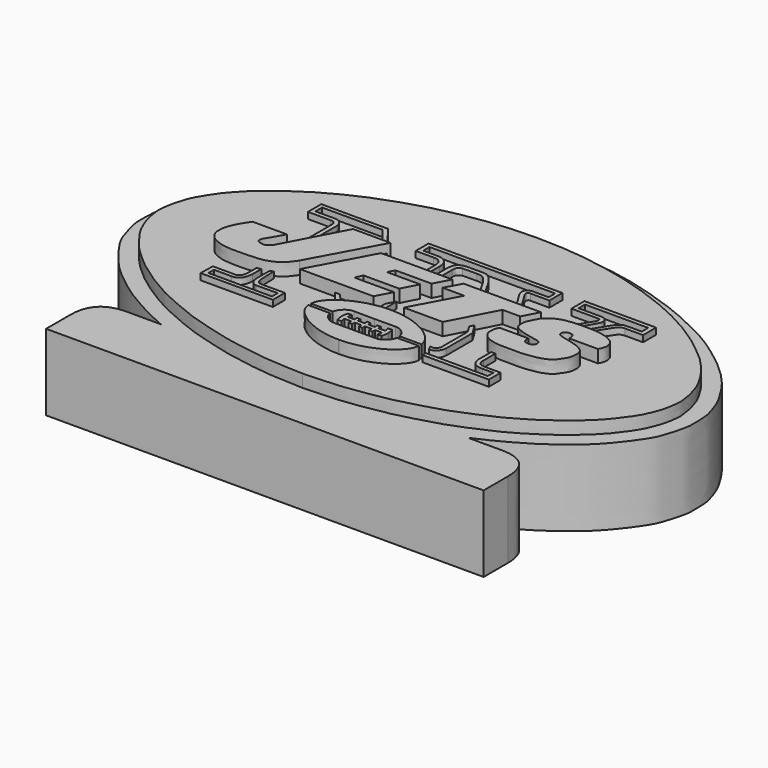
from build123d import *

# Parameters (mm, degrees)
F2_DEPTH     = 12
F3_DEPTH     = 14
F5_DEPTH     = 15
F7_DEPTH     = 4
F9_DEPTH     = 4
F10_T1_DEPTH = 37


# Not quite as in the source:
# - a fillet or chamfer that OpenCascade refuses, or shapes differently, is made with other operations: its cross-section is extruded or revolved along the edge and cut away or added


with BuildPart() as f2:
    # F1 (on Top) → F2 (new body)
    with BuildSketch(Plane.XY):
        with BuildLine():
            add(Edge.make_bspline(
                [(50.0025562942, 75.6758823991), (50.5734645841, 75.691096263), (51.8255528283, 75.7244625681), (54.4006627956, 75.5977520007), (57.6347750084, 75.2942905591), (61.7349234565, 74.7641274687), (66.1555331278, 73.7004555562), (70.1086951054, 72.4083695898), (73.509978518, 71.2064859809), (76.9068851901, 69.5703275722), (80.5021656452, 67.787433424), (82.7753507887, 66.0884500974), (84.690547997, 64.791957351), (87.2991029331, 62.539802007), (89.474339904, 60.2935357758), (90.8590708908, 58.2023483449), (92.2955378458, 55.9070421261), (93.0454197579, 53.566009378), (93.4789474458, 52.1299201465), (93.4965496129, 50.1283577884), (93.5263939672, 48.7731375152), (93.3052010322, 47.5203555479), (92.4675772987, 44.5464448188), (91.4648399507, 42.5938998196), (88.0046401991, 38.0105737186), (84.8677171897, 35.4808355526), (82.0331102601, 33.3582099907), (78.8452327686, 31.5254525863), (76.1158658946, 30.1179831922), (74.404632505, 29.3878864857), (74.1792457822, 29.2939152569)],
                knots=[0, 0, 0, 0, 0.0226261639, 0.0496226001, 0.0802319329, 0.1147737492, 0.1511081815, 0.1856509076, 0.2176496426, 0.2506916306, 0.2847396848, 0.3129679659, 0.3385973423, 0.3700271745, 0.4001251998, 0.4268498403, 0.4548312793, 0.4811225608, 0.5020158854, 0.5257559212, 0.5452333078, 0.564368343, 0.5933886056, 0.6194132177, 0.65943343, 0.6941761055, 0.7255349494, 0.7577990285, 0.7937753727, 0.7991574142, 0.7991574142, 0.7991574142, 0.7991574142], degree=3))
            add(Edge.make_bspline(
                [(50.0025562942, 75.6758823991), (49.4316480043, 75.691096263), (48.1795597601, 75.7244625681), (45.6044497928, 75.5977520007), (42.37033758, 75.2942905591), (38.2701891319, 74.7641274687), (33.8495794606, 73.7004555562), (29.896417483, 72.4083695898), (26.4951340704, 71.2064859809), (23.0982273983, 69.5703275722), (19.5029469432, 67.787433424), (17.2297617997, 66.0884500974), (15.3145645914, 64.791957351), (12.7060096553, 62.539802007), (10.5307726844, 60.2935357758), (9.1460416976, 58.2023483449), (7.7095747426, 55.9070421261), (6.9596928305, 53.566009378), (6.5261651426, 52.1299201465), (6.5085629755, 50.1283577884), (6.4787186212, 48.7731375152), (6.6999115562, 47.5203555479), (7.5375352897, 44.5464448188), (8.5402726377, 42.5938998196), (12.0004723893, 38.0105737186), (15.1373953987, 35.4808355526), (17.9720023283, 33.3582099907), (21.1598798198, 31.5254525863), (23.8892466938, 30.1179831922), (25.6004800834, 29.3878864857), (25.8258668062, 29.2939152569)],
                knots=[0, 0, 0, 0, 0.0226261639, 0.0496226001, 0.0802319329, 0.1147737492, 0.1511081815, 0.1856509076, 0.2176496426, 0.2506916306, 0.2847396848, 0.3129679659, 0.3385973423, 0.3700271745, 0.4001251998, 0.4268498403, 0.4548312793, 0.4811225608, 0.5020158854, 0.5257559212, 0.5452333078, 0.564368343, 0.5933886056, 0.6194132177, 0.65943343, 0.6941761055, 0.7255349494, 0.7577990285, 0.7937753727, 0.7991574142, 0.7991574142, 0.7991574142, 0.7991574142], degree=3))
            Line((25.8258668062, 29.2939152569), (74.1792457822, 29.2939152569))
        make_face()
        with BuildLine():
            Line((74.1792457822, 29.2939152569), (25.8258668062, 29.2939152569))
            add(Edge.make_bspline(
                [(25.8258668062, 29.2939152569), (27.2908028019, 28.6831346664), (30.6454165682, 27.4786700415), (35.7062683791, 26.036881278), (39.3620291273, 25.2816885131), (45.2819531527, 24.5211502985), (47.6329385812, 24.3692576932), (49.220878771, 24.4032193557), (50.0025562942, 24.4199372828)],
                knots=[0.7991574142, 0.7991574142, 0.7991574142, 0.7991574142, 0.8341388289, 0.8734744658, 0.9071846207, 0.9480415389, 0.9744229906, 1, 1, 1, 1], degree=3))
            add(Edge.make_bspline(
                [(74.1792457822, 29.2939152569), (72.7143097865, 28.6831346664), (69.3596960202, 27.4786700415), (64.2988442093, 26.036881278), (60.6430834611, 25.2816885131), (54.7231594357, 24.5211502985), (52.3721740072, 24.3692576932), (50.7842338174, 24.4032193557), (50.0025562942, 24.4199372828)],
                knots=[0.7991574142, 0.7991574142, 0.7991574142, 0.7991574142, 0.8341388289, 0.8734744658, 0.9071846207, 0.9480415389, 0.9744229906, 1, 1, 1, 1], degree=3))
        make_face()
        with BuildLine():
            add(Edge.make_bspline(
                [(25.8258668062, 29.2939152569), (27.2908028019, 28.6831346664), (30.6454165682, 27.4786700415), (35.7062683791, 26.036881278), (39.3620291273, 25.2816885131), (45.2819531527, 24.5211502985), (47.6329385812, 24.3692576932), (49.220878771, 24.4032193557), (50.0025562942, 24.4199372828)],
                knots=[0.7991574142, 0.7991574142, 0.7991574142, 0.7991574142, 0.8341388289, 0.8734744658, 0.9071846207, 0.9480415389, 0.9744229906, 1, 1, 1, 1], degree=3))
            Line((25.8258668062, 29.2939152569), (15.5581459403, 29.2939152569))
            Line((15.5581459403, 29.2939152569), (15.5581459403, 19.5459593087))
            Line((15.5581459403, 19.5459593087), (84.4469666481, 19.5459593087))
            Line((84.4469666481, 19.5459593087), (84.4469666481, 29.2939152569))
            Line((84.4469666481, 29.2939152569), (74.1792457822, 29.2939152569))
            add(Edge.make_bspline(
                [(74.1792457822, 29.2939152569), (72.7143097865, 28.6831346664), (69.3596960202, 27.4786700415), (64.2988442093, 26.036881278), (60.6430834611, 25.2816885131), (54.7231594357, 24.5211502985), (52.3721740072, 24.3692576932), (50.7842338174, 24.4032193557), (50.0025562942, 24.4199372828)],
                knots=[0.7991574142, 0.7991574142, 0.7991574142, 0.7991574142, 0.8341388289, 0.8734744658, 0.9071846207, 0.9480415389, 0.9744229906, 1, 1, 1, 1], degree=3))
        make_face()
    extrude(amount=F2_DEPTH)

    # F0 (on Top) → F3 (join)
    with BuildSketch(Plane.XY):
        with BuildLine():
            add(Edge.make_bspline(
                [(50, 73.1647089124), (51.1726790007, 73.1447049127), (53.3541351944, 73.1074928119), (55.8957948393, 72.8947316687), (58.7288666129, 72.584027711), (62.6788773277, 71.8549312996), (65.8762167839, 71.074486134), (68.8854108818, 70.1422565295), (72.1644056269, 68.9381535509), (74.5103434742, 67.9402710371), (77.2525854937, 66.5636259529), (79.116511075, 65.4990426429), (81.042200528, 64.2345095166), (82.7219046772, 63.0355801846), (84.017534796, 61.911301514), (85.6963281143, 60.6126679604), (86.6881458316, 59.4189416785), (87.6723169201, 58.4199860872), (88.6040772004, 57.0368352742), (89.1222990133, 56.1834449044), (89.6450524555, 55.3026620019), (90.1305801299, 54.2908390403), (90.387367758, 53.3198103837), (90.7344362409, 52.3223687563), (90.8507798363, 51.1606605075), (91.0817424918, 50.0474842463), (90.8762163167, 48.6176411096), (90.6179815584, 47.2300640759), (90.1208350497, 45.8763864159), (89.4898369203, 44.4349683639), (88.688239644, 43.2073573728), (87.9945850029, 42.2936013243), (87.2413523871, 41.2939985832), (86.5652547292, 40.5014768549), (85.6562852165, 39.5740004325), (84.5282435736, 38.5676229102), (83.4762134102, 37.6306351881), (82.3676425163, 36.7978793114), (81.0561736571, 35.8605046963), (79.7202316779, 34.9654467093), (78.2341260878, 34.0977752604), (76.8455245855, 33.2817286477), (75.3374457617, 32.5793308239), (73.7222449823, 31.870879127), (71.6869509536, 30.9944710602), (69.3707514859, 30.102308225), (66.2300657416, 29.2420926336), (63.1930305885, 28.3848585744), (60.1488991033, 27.8606664455), (56.751175539, 27.3019586268), (53.5613273302, 27.0781826454), (50.2328289556, 26.9301487139), (50.0370268982, 26.9425493392), (50, 26.9448943436)],
                knots=[0, 0, 0, 0, 0.0262420027, 0.0488162398, 0.0728641506, 0.1015146266, 0.1275181373, 0.1529026379, 0.1793849828, 0.2025018741, 0.2272210344, 0.2483296919, 0.2698867919, 0.2903049178, 0.3091212763, 0.3298178208, 0.347556948, 0.364527844, 0.3828522247, 0.3971672122, 0.4114750851, 0.4265799493, 0.4408750286, 0.4554926872, 0.4708277084, 0.4860229221, 0.5030499454, 0.5200612326, 0.5371645352, 0.5551420039, 0.5723581176, 0.5877158735, 0.6035254716, 0.6181001876, 0.6342917892, 0.651928954, 0.6688550771, 0.6856305129, 0.7037034691, 0.7218953267, 0.7405834267, 0.7587203624, 0.7770021848, 0.7959530968, 0.8170538963, 0.8396335302, 0.8653946001, 0.890826804, 0.9159033542, 0.9420696145, 0.9691025611, 0.9941571793, 1, 1, 1, 1], degree=3))
            add(Edge.make_bspline(
                [(50, 73.1647089124), (48.8273209993, 73.1447049127), (46.6458648056, 73.1074928119), (44.1042051607, 72.8947316687), (41.2711333871, 72.584027711), (37.3211226723, 71.8549312996), (34.1237832161, 71.074486134), (31.1145891182, 70.1422565295), (27.8355943731, 68.9381535509), (25.4896565258, 67.9402710371), (22.7474145063, 66.5636259529), (20.883488925, 65.4990426429), (18.957799472, 64.2345095166), (17.2780953228, 63.0355801846), (15.982465204, 61.911301514), (14.3036718857, 60.6126679604), (13.3118541684, 59.4189416785), (12.3276830799, 58.4199860872), (11.3959227996, 57.0368352742), (10.8777009867, 56.1834449044), (10.3549475445, 55.3026620019), (9.8694198701, 54.2908390403), (9.612632242, 53.3198103837), (9.2655637591, 52.3223687563), (9.1492201637, 51.1606605075), (8.9182575082, 50.0474842463), (9.1237836833, 48.6176411096), (9.3820184416, 47.2300640759), (9.8791649503, 45.8763864159), (10.5101630797, 44.4349683639), (11.311760356, 43.2073573728), (12.0054149971, 42.2936013243), (12.7586476129, 41.2939985832), (13.4347452708, 40.5014768549), (14.3437147835, 39.5740004325), (15.4717564264, 38.5676229102), (16.5237865898, 37.6306351881), (17.6323574837, 36.7978793114), (18.9438263429, 35.8605046963), (20.2797683221, 34.9654467093), (21.7658739122, 34.0977752604), (23.1544754145, 33.2817286477), (24.6625542383, 32.5793308239), (26.2777550177, 31.870879127), (28.3130490464, 30.9944710602), (30.6292485141, 30.102308225), (33.7699342584, 29.2420926336), (36.8069694115, 28.3848585744), (39.8511008967, 27.8606664455), (43.248824461, 27.3019586268), (46.4386726698, 27.0781826454), (49.7671710444, 26.9301487139), (49.9629731018, 26.9425493392), (50, 26.9448943436)],
                knots=[0, 0, 0, 0, 0.0262420027, 0.0488162398, 0.0728641506, 0.1015146266, 0.1275181373, 0.1529026379, 0.1793849828, 0.2025018741, 0.2272210344, 0.2483296919, 0.2698867919, 0.2903049178, 0.3091212763, 0.3298178208, 0.347556948, 0.364527844, 0.3828522247, 0.3971672122, 0.4114750851, 0.4265799493, 0.4408750286, 0.4554926872, 0.4708277084, 0.4860229221, 0.5030499454, 0.5200612326, 0.5371645352, 0.5551420039, 0.5723581176, 0.5877158735, 0.6035254716, 0.6181001876, 0.6342917892, 0.651928954, 0.6688550771, 0.6856305129, 0.7037034691, 0.7218953267, 0.7405834267, 0.7587203624, 0.7770021848, 0.7959530968, 0.8170538963, 0.8396335302, 0.8653946001, 0.890826804, 0.9159033542, 0.9420696145, 0.9691025611, 0.9941571793, 1, 1, 1, 1], degree=3))
        make_face()
    extrude(amount=F3_DEPTH)

    # F4 (on Top) → F5 (join)
    with BuildSketch(Plane.XY):
        with BuildLine():
            Line((24.8472932726, 62.0919987559), (24.8472932726, 62.0547011495))
            Line((24.8472932726, 62.0547011495), (24.8472932726, 59.4672113657))
            Line((24.8472932726, 59.4672113657), (28.432648629, 59.4672113657))
            add(Edge.make_bspline(
                [(28.432648629, 59.4672113657), (28.5770956375, 59.4680223715), (28.8478765215, 59.4695426858), (29.0899402402, 59.2343324012), (29.1894485193, 59.0413391973), (29.2421844006, 58.8522367885), (29.2483326023, 58.6431159146), (29.2518343776, 58.5240088403)],
                knots=[0, 0, 0, 0, 0.2395232585, 0.4490111659, 0.6208103722, 0.7840284123, 1, 1, 1, 1], degree=3))
            Line((29.2518343776, 58.5240088403), (29.2518343776, 51.8394894898))
            Line((29.2518343776, 51.8394894898), (29.950324446, 52.9840327799))
            Line((29.950324446, 52.9840327799), (29.950324446, 58.7685331702))
            add(Edge.make_bspline(
                [(29.950324446, 58.7685331702), (29.9219447597, 58.9523760844), (29.8624838947, 59.3375621161), (29.4687268151, 59.9229242198), (28.8248198348, 60.1495592762), (28.5701259956, 60.1478221831), (28.4624826163, 60.147088021)],
                knots=[0, 0, 0, 0, 0.2528176638, 0.5297013112, 0.8012337468, 1, 1, 1, 1], degree=3))
            Line((28.4624826163, 60.147088021), (25.4870709032, 60.147088021))
            Line((25.4870709032, 60.147088021), (25.4870709032, 61.4588186145))
            Line((25.4870709032, 61.4588186145), (35.027064383, 61.4588186145))
            Line((35.027064383, 61.4588186145), (37.3411662877, 58.4819130599))
            Line((37.3411662877, 58.4819130599), (38.1168499589, 58.4819130599))
            Line((38.1168499589, 58.4819130599), (35.3702530265, 62.0919987559))
            Line((35.3702530265, 62.0919987559), (24.8472932726, 62.0919987559))
        make_face()
        Polygon((31.8974405527, 56.6574372351), (30.9292972088, 57.7732659876), (30.9292972088, 54.9016445875), align=None)
        Polygon((40.307242797, 55.6674497355), (39.3718518317, 56.8707548082), (38.993286447, 56.2599888853), (39.4538976252, 55.6674497355), align=None)
        with BuildLine():
            Line((29.893040657, 43.9803116024), (29.3342024088, 43.9044199884))
            Line((29.3342024088, 43.9044199884), (29.2301792651, 43.8636392355))
            Line((29.2301792651, 43.8636392355), (29.2301792651, 42.2408729792))
            add(Edge.make_bspline(
                [(28.4447427839, 40.8443361521), (28.5288231599, 40.8693041169), (28.7135275939, 40.9241527515), (29.0226877497, 41.1991019599), (29.1709378952, 41.6794222452), (29.2099592207, 42.0492406994), (29.2301792651, 42.2408729792)],
                knots=[0, 0, 0, 0, 0.2003141152, 0.4400421006, 0.7098413893, 1, 1, 1, 1], degree=3))
            Line((28.4447427839, 40.8443361521), (24.7761104256, 40.8443361521))
            Line((24.7761104256, 40.8443361521), (24.7224476188, 38.4893082082))
            Line((24.7224476188, 38.4893082082), (36.1039862037, 38.4893082082))
            Line((36.1039862037, 38.4893082082), (36.1039862037, 40.8443361521))
            Line((36.1039862037, 40.8443361521), (32.6897762716, 40.8443361521))
            add(Edge.make_bspline(
                [(31.5591432154, 41.8013744056), (31.5841833672, 41.689429146), (31.6343731368, 41.4650492451), (31.7628271947, 41.135785545), (32.0783227272, 40.8327697797), (32.472171476, 40.8402198981), (32.6897762716, 40.8443361521)],
                knots=[0, 0, 0, 0, 0.2271778453, 0.4553488251, 0.6990755767, 1, 1, 1, 1], degree=3))
            Line((31.5591432154, 41.8013744056), (31.4688906074, 44.4679968059))
            Line((31.4688906074, 44.4679968059), (30.9789907187, 44.2300625145))
            Line((30.9789907187, 44.2300625145), (30.9789907187, 41.8013744056))
            add(Edge.make_bspline(
                [(32.0542082191, 40.2117855847), (31.9064026604, 40.2584518208), (31.6114569709, 40.3515741994), (31.2394463911, 40.6616765722), (31.0556805424, 41.1210527513), (31.0060815614, 41.5610493397), (30.9789907187, 41.8013744056)],
                knots=[0, 0, 0, 0, 0.2361364432, 0.4712097888, 0.7111760734, 1, 1, 1, 1], degree=3))
            Line((32.0542082191, 40.2117855847), (35.4624316096, 40.2523949742))
            Line((35.4624316096, 40.2523949742), (35.4624316096, 39.1094908118))
            Line((35.4624316096, 39.1094908118), (25.450931862, 39.1094908118))
            Line((25.450931862, 39.1094908118), (25.450931862, 40.2117855847))
            Line((25.450931862, 40.2117855847), (28.2472763211, 40.2117855847))
            add(Edge.make_bspline(
                [(29.893040657, 42.29689762), (29.8729205699, 42.0992567369), (29.8328819333, 41.7059546897), (29.6610606398, 41.1466974039), (29.4056773273, 40.641042287), (28.934915075, 40.345353847), (28.7008461081, 40.2321347606), (28.4117523205, 40.2191647161), (28.2472763211, 40.2117855847)],
                knots=[0, 0, 0, 0, 0.183915353, 0.3659884724, 0.5457499936, 0.7190014354, 0.8401296683, 1, 1, 1, 1], degree=3))
            Line((29.893040657, 42.29689762), (29.893040657, 43.9803116024))
        make_face()
        Polygon((41.6667759418, 44.7726286948), (40.8699139953, 44.7726286948), (42.9920303253, 42.1391799425), (43.5088723898, 42.5717718899), align=None)
        Polygon((48.2891350985, 44.3227551877), (48.2891350985, 47.6205907762), (47.5578159094, 46.3166348636), (47.5578159094, 44.2300625145), align=None)
        with BuildLine():
            Line((62.7717524767, 62.1425397694), (41.7551808059, 62.1425397694))
            Line((41.7551808059, 62.1425397694), (41.6903570294, 62.1425397694))
            Line((41.6903570294, 62.1425397694), (41.6903570294, 59.6215501428))
            Line((41.6903570294, 59.6215501428), (44.5214621723, 59.6215501428))
            add(Edge.make_bspline(
                [(45.9278970957, 58.2406893373), (45.8958359243, 58.4494538935), (45.8361942703, 58.8378072475), (45.6285011734, 59.2526765072), (45.3158703423, 59.4862073114), (45.0442849958, 59.6244029722), (44.7115516537, 59.622587383), (44.5214621723, 59.6215501428)],
                knots=[0, 0, 0, 0, 0.2348794459, 0.4369334635, 0.619809008, 0.7827981168, 1, 1, 1, 1], degree=3))
            Line((45.9278970957, 58.2406893373), (45.9278970957, 55.6644387543))
            Line((45.9278970957, 55.6644387543), (45.9812283516, 55.6644387543))
            Line((45.9812283516, 55.6644387543), (46.5663038194, 55.6644387543))
            Line((46.5663038194, 55.6644387543), (46.5663038194, 58.20755288))
            add(Edge.make_bspline(
                [(44.9001155794, 60.2544024587), (45.0649355324, 60.2248855618), (45.3920799421, 60.1662986758), (45.8350689766, 59.9682432593), (46.2141152844, 59.5334912824), (46.4304248795, 59.1994293791), (46.5473114118, 58.6680528417), (46.5601060574, 58.3578270973), (46.5663038194, 58.20755288)],
                knots=[0, 0, 0, 0, 0.1681834258, 0.3338204297, 0.5122773709, 0.6638179796, 0.8371524902, 1, 1, 1, 1], degree=3))
            Line((44.9001155794, 60.2544024587), (42.368169874, 60.2544024587))
            Line((42.368169874, 60.2544024587), (42.368169874, 61.4935383201))
            Line((42.368169874, 61.4935383201), (62.1532574296, 61.4935383201))
            Line((62.1532574296, 61.4935383201), (62.1532574296, 60.2030679584))
            Line((62.1532574296, 60.2030679584), (59.9544197321, 60.2030679584))
            add(Edge.make_bspline(
                [(58.932941407, 58.4308691323), (58.8622270321, 58.5867351514), (58.7268858777, 58.8850491365), (58.5869951488, 59.2822181909), (58.6991143843, 59.7306100989), (58.9319145846, 59.9244223305), (59.3358866975, 60.2166880772), (59.7390002219, 60.2078115034), (59.9544197321, 60.2030679584)],
                knots=[0, 0, 0, 0, 0.1761985529, 0.3372286838, 0.4988354932, 0.6341869223, 0.8045134454, 1, 1, 1, 1], degree=3))
            Line((58.932941407, 58.4308691323), (60.6204718351, 55.7104982436))
            Line((60.6204718351, 55.7104982436), (61.3897368312, 55.7104982436))
            Line((61.3897368312, 55.7104982436), (59.5662333071, 58.6588159204))
            add(Edge.make_bspline(
                [(59.795871377, 59.5764480531), (59.7358157798, 59.5866663442), (59.6029907603, 59.609266148), (59.3594082086, 59.4097176123), (59.3798910003, 59.1055065904), (59.4367107896, 58.8447315758), (59.5244288267, 58.7188217597), (59.5662333071, 58.6588159204)],
                knots=[0, 0, 0, 0, 0.1735648204, 0.3838734725, 0.6014923928, 0.81008007, 1, 1, 1, 1], degree=3))
            Line((59.795871377, 59.5764480531), (62.7717524767, 59.5764480531))
            Line((62.7717524767, 59.5764480531), (62.7717524767, 62.1425397694))
        make_face()
        with BuildLine():
            Line((47.566100955, 58.5536807775), (47.566100955, 55.6644387543))
            Line((47.566100955, 55.6644387543), (48.3492165804, 55.6644387543))
            Line((48.3492165804, 55.6644387543), (48.3492165804, 58.4910288453))
            add(Edge.make_bspline(
                [(48.3492165804, 58.4910288453), (48.3479479164, 58.5479872156), (48.3449691962, 58.6817208597), (48.3713964371, 59.0449616758), (48.5236488183, 59.2190359266), (48.779307881, 59.4672298691), (48.9881080981, 59.5341711855), (49.0912869573, 59.5672503114)],
                knots=[0, 0, 0, 0, 0.1640944248, 0.3852804302, 0.5655773907, 0.7853295852, 1, 1, 1, 1], degree=3))
            Line((49.0912869573, 59.5672503114), (51.4055304229, 59.5858767629))
            add(Edge.make_bspline(
                [(53.3237680793, 58.3565793931), (53.2367182753, 58.4724054285), (53.0608695058, 58.7063848844), (52.7924904462, 59.0501999123), (52.3876924541, 59.4036361084), (52.1107435217, 59.5023577213), (51.8573160762, 59.5861824228), (51.5699599356, 59.5859880092), (51.4055304229, 59.5858767629)],
                knots=[0, 0, 0, 0, 0.1743242869, 0.3521514115, 0.5450254676, 0.6867589695, 0.8207587633, 1, 1, 1, 1], degree=3))
            Line((53.3237680793, 58.3565793931), (54.8743344843, 55.6704998016))
            Line((54.8743344843, 55.6704998016), (55.602632463, 55.6704998016))
            Line((55.602632463, 55.6704998016), (54.1068837047, 58.3565793931))
            add(Edge.make_bspline(
                [(52.0160868764, 60.276158154), (52.1441648745, 60.2499349732), (52.4146192643, 60.1945611036), (52.8406581336, 59.9243022626), (53.223901683, 59.5411266774), (53.6440666457, 59.0848234251), (53.943922428, 58.6129994512), (54.1068837047, 58.3565793931)],
                knots=[0, 0, 0, 0, 0.1668660601, 0.3523607422, 0.5460428535, 0.7532899464, 1, 1, 1, 1], degree=3))
            Line((52.0160868764, 60.276158154), (49.2733605206, 60.276158154))
            add(Edge.make_bspline(
                [(47.566100955, 58.5536807775), (47.6017111637, 58.7501406209), (47.6715287166, 59.1353207701), (47.7979462105, 59.68373798), (48.298332696, 60.0880836096), (48.7501313722, 60.1995135762), (49.0582668137, 60.2801389796), (49.2066058623, 60.2773936093), (49.2733605206, 60.276158154)],
                knots=[0, 0, 0, 0, 0.193156866, 0.3787043154, 0.5743968463, 0.7461992779, 0.8857861053, 1, 1, 1, 1], degree=3))
        make_face()
        with BuildLine():
            Line((66.2426501513, 62.1425397694), (66.2426501513, 59.5764480531))
            Line((66.2426501513, 59.5764480531), (70.4862996936, 59.5833994448))
            add(Edge.make_bspline(
                [(70.7050338387, 58.9078292251), (70.7203915835, 58.9557411557), (70.755797534, 59.0661979627), (70.7507253504, 59.3367151233), (70.7403095201, 59.5535032349), (70.5740284121, 59.5730740325), (70.4862996936, 59.5833994448)],
                knots=[0, 0, 0, 0, 0.219800406, 0.506730802, 0.7397547132, 1, 1, 1, 1], degree=3))
            Line((70.7050338387, 58.9078292251), (68.8942819834, 55.8677688241))
            Line((68.8942819834, 55.8677688241), (69.6806013584, 55.8677688241))
            add(Edge.make_bspline(
                [(70.5936178565, 60.212995857), (70.6975565997, 60.1966138847), (70.906059749, 60.1637513281), (71.171838004, 59.9792846266), (71.3788683088, 59.6545238798), (71.4567593115, 59.3603453525), (71.4367845884, 59.0278623136), (71.3317045555, 58.6785807243), (70.3968660645, 57.0871265015), (69.6806013584, 55.8677688241)],
                knots=[0, 0, 0, 0, 0.1068915044, 0.2144264462, 0.3320753563, 0.4385488739, 0.5434327776, 0.6501823679, 1, 1, 1, 1], degree=3))
            Line((70.5936178565, 60.212995857), (66.859818995, 60.212995857))
            Line((66.859818995, 60.212995857), (66.859818995, 61.4773519337))
            Line((66.859818995, 61.4773519337), (76.8100246787, 61.4773519337))
            Line((76.8100246787, 61.4773519337), (76.8100246787, 60.212995857))
            Line((76.8100246787, 60.212995857), (75.1242190599, 60.212995857))
            add(Edge.make_bspline(
                [(72.8391632438, 59.0803474188), (72.937538574, 59.22475605), (73.1372931249, 59.5179828294), (73.5618770133, 59.8810052536), (73.990662846, 60.1859666784), (74.5062244077, 60.2107864204), (74.9105586426, 60.2122319845), (75.1242190599, 60.212995857)],
                knots=[0, 0, 0, 0, 0.1970439725, 0.4001046819, 0.5936394596, 0.7852688317, 1, 1, 1, 1], degree=3))
            Line((72.8391632438, 59.0803474188), (70.9558054805, 55.9637658298))
            Line((70.9558054805, 55.9637658298), (71.6853067279, 55.9637658298))
            add(Edge.make_bspline(
                [(74.6454671025, 59.5764480531), (74.5556534601, 59.5714437324), (74.3579936706, 59.5604303388), (73.9435226211, 59.3764107664), (73.5403079468, 58.9740526599), (72.4668413174, 57.2320363076), (71.6853067279, 55.9637658298)],
                knots=[0, 0, 0, 0, 0.1407859289, 0.3098384199, 0.4975296553, 1, 1, 1, 1], degree=3))
            Line((74.6454671025, 59.5764480531), (77.5194913149, 59.5764480531))
            Line((77.5194913149, 59.5764480531), (77.5194913149, 62.1425397694))
            Line((77.5194913149, 62.1425397694), (66.2426501513, 62.1425397694))
        make_face()
        with BuildLine():
            Line((60.8194805682, 46.8982756138), (59.7332790494, 48.6643537879))
            Line((59.7332790494, 48.6643537879), (59.3776777387, 48.045348376))
            Line((59.3776777387, 48.045348376), (60.1481460035, 46.7875786126))
            Line((60.1481460035, 46.7875786126), (60.1481460035, 41.8338961899))
            add(Edge.make_bspline(
                [(60.1481460035, 41.8338961899), (60.1425823617, 41.6802548204), (60.1324046433, 41.3991945641), (59.9581751903, 41.1406898924), (59.7324820562, 40.9710311689), (59.5513266598, 40.8460640868), (59.2733342443, 40.8658433556), (59.0861996953, 40.8586630306), (58.9907765388, 40.8550016582)],
                knots=[0, 0, 0, 0, 0.2030782532, 0.3714964666, 0.5338819123, 0.675412732, 0.834487315, 1, 1, 1, 1], degree=3))
            Line((58.9907765388, 40.8550016582), (59.3185387552, 40.1838682592))
            add(Edge.make_bspline(
                [(60.8194805682, 41.6709184647), (60.7909169812, 41.4913387017), (60.7324261477, 41.1236058236), (60.4096326152, 40.6020811333), (59.9400189384, 40.2176569594), (59.5273989164, 40.1952235905), (59.3185387552, 40.1838682592)],
                knots=[0, 0, 0, 0, 0.24217256, 0.4959067268, 0.7448378734, 1, 1, 1, 1], degree=3))
            Line((60.8194805682, 41.6709184647), (60.8194805682, 46.8982756138))
        make_face()
        with BuildLine():
            Line((69.4123357534, 39.1423292458), (59.6617795527, 39.1609556973))
            Line((59.6617795527, 39.1609556973), (59.6617795527, 38.4904295206))
            Line((59.6617795527, 38.4904295206), (70.1107978821, 38.4904295206))
            Line((70.1107978821, 38.4904295206), (70.1107978821, 40.8279560506))
            Line((70.1107978821, 40.8279560506), (67.3914477229, 40.8279560506))
            add(Edge.make_bspline(
                [(67.3914477229, 40.8279560506), (67.2361362215, 40.8485982808), (66.9221810351, 40.8903256169), (66.5689572315, 41.256496478), (66.418769631, 41.6969626993), (66.421576881, 41.9539069874), (66.4229094982, 42.0758798718)],
                knots=[0, 0, 0, 0, 0.2553149594, 0.5161076607, 0.7702936118, 1, 1, 1, 1], degree=3))
            Line((66.4229094982, 42.0758798718), (66.4229094982, 44.3947762251))
            Line((66.4229094982, 44.3947762251), (65.7617002726, 44.3947762251))
            Line((65.7617002726, 44.3947762251), (65.7617002726, 41.7592376471))
            add(Edge.make_bspline(
                [(65.7617002726, 41.7592376471), (65.8089255178, 41.5760040169), (65.9007665282, 41.2196615218), (66.1645750586, 40.7750808042), (66.4017224691, 40.5381065359), (66.7799530774, 40.3850049548), (67.2569170834, 40.2185216991), (67.5492340077, 40.2401726311), (67.6894560456, 40.2505584061)],
                knots=[0, 0, 0, 0, 0.1867230908, 0.3631286026, 0.5041834475, 0.6612195099, 0.8374897695, 1, 1, 1, 1], degree=3))
            Line((67.6894560456, 40.2505584061), (69.4123357534, 40.2505584061))
            Line((69.4123357534, 40.2505584061), (69.4123357534, 39.1423292458))
        make_face()
    extrude(amount=F5_DEPTH)

    # F6 (on face) → F7 (join)
    with BuildSketch(Plane.XY.offset(12)):
        with BuildLine():
            Line((39.1289107502, 57.861559093), (33.2370586693, 57.861559093))
            Line((33.2370586693, 57.861559093), (28.3640995622, 48.6583039165))
            add(Edge.make_bspline(
                [(28.3640995622, 48.6583039165), (28.3035658947, 48.5465067942), (28.1773181568, 48.3133450778), (27.8190698766, 48.0234016095), (27.453452225, 47.7743981871), (26.9666919945, 47.7917733347), (26.6197609632, 47.8544715233), (26.2972630041, 47.9449034128), (26.1194592224, 48.138413903), (26.0301029724, 48.4074772023), (26.0986608017, 48.8018753786), (26.408180621, 49.2500716599), (27.2200654772, 50.6669416881), (27.7932640165, 51.667265594)],
                knots=[0, 0, 0, 0, 0.0794521811, 0.1657037904, 0.2500781313, 0.337353949, 0.4144472779, 0.4868883847, 0.5504236145, 0.6171634067, 0.6936878923, 0.7837406975, 1, 1, 1, 1], degree=3))
            Line((27.7932640165, 51.667265594), (22.4987771362, 51.667265594))
            Line((22.4987771362, 51.667265594), (22.3526973277, 51.667265594))
            add(Edge.make_bspline(
                [(22.3526973277, 51.667265594), (22.2534780363, 51.5224875309), (22.0441133542, 51.216988341), (21.6906398426, 50.6458276522), (21.3548615035, 50.0984386414), (21.0555368856, 49.4605332408), (20.7552602813, 48.8054706373), (20.5379539174, 47.8866039297), (20.5767154609, 47.3082667964), (20.521310261, 46.7772970904), (20.7537594928, 46.2013664118), (21.0383951709, 45.8160868942), (21.6150443102, 45.1581029622), (22.2657033556, 44.8977953885), (23.2231252253, 44.4926831325), (23.8546044511, 44.4613136286), (24.6514855532, 44.3206369341), (25.7776390284, 44.3069619846), (26.9340743057, 44.3057278672), (27.9570342358, 44.3987567643), (29.0770404873, 44.3918629896), (30.2175538903, 44.6490005612), (31.0508076929, 44.9744115826), (32.1464146348, 45.6040959866), (32.6252595787, 46.246966668), (33.0842182462, 46.8032044052), (33.251297229, 47.0753134459), (33.3256572485, 47.196418047)],
                knots=[0, 0, 0, 0, 0.0331907152, 0.0700364156, 0.1063461736, 0.1437507684, 0.1825391749, 0.2260238794, 0.2603281383, 0.2928280334, 0.3273603284, 0.3591207764, 0.4001428196, 0.4387283325, 0.4840207925, 0.5198506608, 0.5597285695, 0.6078351656, 0.6564816781, 0.7020415367, 0.7498421272, 0.7980028787, 0.8412763871, 0.8911699207, 0.9319584716, 0.9697174995, 1, 1, 1, 1], degree=3))
            Line((33.3256572485, 47.196418047), (39.1289107502, 57.861559093))
        make_face()
        Polygon((51.1735826731, 54.9981184304), (39.9260930717, 54.9981184304), (34.7896516323, 45.449603349), (46.3664010167, 45.449603349), (47.6702675223, 47.8729493916), (41.4143465459, 47.8729493916), (41.9675000012, 49.0187741816), (47.5912429392, 49.0187741816), (48.8819405437, 51.5079721808), (43.65330562, 51.5079721808), (44.1669486463, 52.5352619588), (49.8565472662, 52.5352619588), align=None)
        Polygon((65.1248320937, 54.9981184304), (52.9422424734, 54.9981184304), (51.5988655388, 52.5352619588), (55.0099872053, 52.5352619588), (51.1735826731, 45.4348959029), (57.2884604335, 45.4348959029), (61.0288456082, 52.5352619588), (63.8077929616, 52.5352619588), align=None)
        with BuildLine():
            Line((68.1906193495, 48.5900789499), (63.7052804232, 48.5900789499))
            add(Edge.make_bspline(
                [(63.7052804232, 48.5900789499), (63.646887073, 48.4639655583), (63.5224055094, 48.1951200113), (63.3991305249, 47.635685681), (63.3973880073, 47.1967333203), (63.4278423451, 46.5655066664), (63.7565132045, 46.1439324117), (64.0443586746, 45.7750963503), (64.7971061197, 45.3460265947), (65.3146526387, 45.2042121078), (66.2987564946, 44.9640282649), (67.6636922603, 44.9826124328), (69.0908855118, 44.9458618147), (70.2028429557, 44.957805916), (71.572555207, 45.1433707087), (72.5584763688, 45.3278434625), (73.4801212178, 45.6550341117), (74.2773473625, 46.1063943469), (74.7896288451, 46.8656654164), (75.3525563363, 47.6649124011), (75.5267295144, 48.5285688635), (75.541144252, 49.3915849956), (75.301544247, 49.9749969415), (74.8869090422, 50.3287105839), (74.2673923531, 50.7027300378), (73.644061702, 50.9175834415), (72.7220626267, 51.2040109704), (71.8533053168, 51.3835400073), (71.1362337366, 51.5540159812), (70.5752578854, 51.7709257544), (70.4879094601, 52.375401314), (70.7706218727, 52.7327957564), (71.0985615752, 52.8413974386), (71.5073452353, 52.8523452953), (71.8115180564, 52.7938504873), (72.0571753044, 52.55286651), (72.1804230005, 52.2180157543), (72.1908329241, 51.9025289784), (72.1964836121, 51.7312772572)],
                knots=[0, 0, 0, 0, 0.0220508337, 0.0470074461, 0.0695376667, 0.0956093163, 0.1194691441, 0.1425391113, 0.1729618334, 0.1977975284, 0.230645288, 0.2702799741, 0.3101257078, 0.3456839212, 0.3846772988, 0.4184139563, 0.4511778974, 0.4827409267, 0.5145455482, 0.5473982554, 0.57872177, 0.6096002805, 0.6353903032, 0.6597631107, 0.6878394851, 0.7152048843, 0.7479519004, 0.7797984981, 0.8086174867, 0.833298949, 0.8574169036, 0.878999274, 0.8983698129, 0.9196016548, 0.9379964251, 0.9568578567, 0.9765816926, 1, 1, 1, 1], degree=3))
            Line((72.1964836121, 51.7312772572), (76.6876488924, 51.7312772572))
            add(Edge.make_bspline(
                [(76.6876488924, 51.7312772572), (76.7526597203, 51.8434237925), (76.884059626, 52.0700944047), (77.0193880158, 52.4517525338), (77.1237727932, 52.9534521421), (77.0582147947, 53.4805909544), (76.8056023574, 54.0414110843), (76.2378048374, 54.552959265), (75.1985984952, 55.0257919087), (73.8244670013, 55.3176789718), (72.3517782927, 55.3810450572), (70.5101758418, 55.3541262162), (69.1583091767, 55.2460511404), (67.5291263735, 54.886632302), (66.1030136158, 53.769228809), (65.7666421541, 52.8805450152), (65.126454098, 51.8518689942), (65.1431392418, 50.9659896303), (65.2163026105, 50.3280837385), (65.6386504703, 49.8898830512), (66.6780879346, 49.4554261287), (67.6453890847, 49.2028783781), (68.8269271635, 48.9445439986), (69.5832208535, 48.8531767492), (69.8778535708, 48.5794727409), (69.9493300067, 48.3143612534), (70.0074519462, 47.9529308982), (69.689830965, 47.7166344813), (69.4796582326, 47.5107100912), (69.1042830967, 47.4929822432), (68.7316247137, 47.529506182), (68.4842353859, 47.6094148529), (68.3368012018, 47.8801058621), (68.2352940852, 48.1870171768), (68.3148320756, 48.6299061372), (68.2200671418, 48.5995209997), (68.1906193495, 48.5900789499)],
                knots=[0, 0, 0, 0, 0.0222114916, 0.0448938738, 0.0702524691, 0.0961047318, 0.1235281005, 0.1541772025, 0.1921223356, 0.234291318, 0.2781006753, 0.3262694714, 0.3680252521, 0.4140579468, 0.4609127466, 0.4957751029, 0.5343273314, 0.5677311114, 0.5953396511, 0.6221087155, 0.659494402, 0.6961349795, 0.7355662956, 0.7664103157, 0.7875269623, 0.8060741172, 0.826545833, 0.8480513226, 0.867242084, 0.8886270708, 0.9106842656, 0.9282502798, 0.9471455411, 0.9686184217, 0.9902483106, 1, 1, 1, 1], degree=3))
        make_face()
    extrude(amount=F7_DEPTH)

    # F8 (on face) → F9 (join)
    with BuildSketch(Plane.XY.offset(12)):
        with BuildLine():
            add(Edge.make_bspline(
                [(41.5828339756, 39.1416177154), (41.6038977127, 39.2989410762), (41.6484758959, 39.6318919449), (41.8857727592, 40.1879638275), (42.2807758919, 40.7815902995), (42.6903328224, 41.2107257947), (43.2301467721, 41.6721113917), (43.9250619703, 42.2075946854), (44.8107510503, 42.7006244977), (45.5382931062, 43.0010285348), (46.6200949066, 43.4692963643), (48.160641653, 43.7647221686), (48.7129038565, 43.8573185221), (49.589937809, 43.9408942595), (50.0558113254, 43.9386920077), (50.2779074013, 43.9376421273)],
                knots=[0, 0, 0, 0, 0.0599618188, 0.1269000328, 0.1994885198, 0.265734133, 0.3375481342, 0.4190435673, 0.505238129, 0.5810818834, 0.6759569788, 0.7829737653, 0.848891274, 0.927961874, 1, 1, 1, 1], degree=3))
            Line((41.5828339756, 39.1416177154), (44.9985675514, 39.1416177154))
            add(Edge.make_bspline(
                [(44.9985675514, 39.1416177154), (45.0053972823, 39.1673108052), (45.0273196163, 39.249781476), (45.1966478978, 39.7404055282), (45.4842866026, 40.1250325412), (45.9576782417, 40.5407995815), (46.267287296, 40.6933016985), (46.6787950484, 40.8469489512), (46.8972958493, 40.8365756062), (46.9987392426, 40.831759572)],
                knots=[0, 0, 0, 0, 0.0733265916, 0.2353665226, 0.402443431, 0.5821737373, 0.7201120026, 0.8700563656, 1, 1, 1, 1], degree=3))
            Line((46.9987392426, 40.831759572), (50.2779074013, 40.8217869699))
            Line((50.2779074013, 40.8217869699), (53.5570755601, 40.831759572))
            add(Edge.make_bspline(
                [(55.5572472513, 39.1416177154), (55.5504175203, 39.1673108052), (55.5284951864, 39.249781476), (55.3591669048, 39.7404055282), (55.0715282, 40.1250325412), (54.598136561, 40.5407995815), (54.2885275066, 40.6933016985), (53.8770197542, 40.8469489512), (53.6585189533, 40.8365756062), (53.5570755601, 40.831759572)],
                knots=[0, 0, 0, 0, 0.0733265916, 0.2353665226, 0.402443431, 0.5821737373, 0.7201120026, 0.8700563656, 1, 1, 1, 1], degree=3))
            Line((55.5572472513, 39.1416177154), (58.9729808271, 39.1416177154))
            add(Edge.make_bspline(
                [(58.9729808271, 39.1416177154), (58.9519170899, 39.2989410762), (58.9073389067, 39.6318919449), (58.6700420434, 40.1879638275), (58.2750389108, 40.7815902995), (57.8654819803, 41.2107257947), (57.3256680306, 41.6721113917), (56.6307528323, 42.2075946854), (55.7450637523, 42.7006244977), (55.0175216964, 43.0010285348), (53.9357198961, 43.4692963643), (52.3951731496, 43.7647221686), (51.8429109461, 43.8573185221), (50.9658769936, 43.9408942595), (50.5000034773, 43.9386920077), (50.2779074013, 43.9376421273)],
                knots=[0, 0, 0, 0, 0.0599618188, 0.1269000328, 0.1994885198, 0.265734133, 0.3375481342, 0.4190435673, 0.505238129, 0.5810818834, 0.6759569788, 0.7829737653, 0.848891274, 0.927961874, 1, 1, 1, 1], degree=3))
        make_face()
        with BuildLine():
            Line((44.9969167757, 38.5988134528), (41.5812463828, 38.6195891101))
            add(Edge.make_bspline(
                [(41.5812463828, 38.6195891101), (41.601352836, 38.4621405425), (41.6439050738, 38.1289246928), (41.8778153287, 37.5714197758), (42.269200516, 36.9754017406), (42.6761397221, 36.5437831183), (43.2131373819, 36.0791227232), (43.9047827337, 35.5394226233), (44.787456655, 35.0410148676), (45.5131580933, 34.7361912282), (46.5920917182, 34.2613521728), (48.1308130876, 33.9565617022), (48.6825018729, 33.8606080142), (49.5590112663, 33.771699403), (50.0248895599, 33.7710680124), (50.2469879134, 33.7707670093)],
                knots=[0, 0, 0, 0, 0.0599618188, 0.1269000328, 0.1994885198, 0.265734133, 0.3375481342, 0.4190435673, 0.505238129, 0.5810818834, 0.6759569788, 0.7829737653, 0.848891274, 0.927961874, 1, 1, 1, 1], degree=3))
            Line((50.2469879134, 33.7707670093), (50.3088268893, 33.7707670093))
            add(Edge.make_bspline(
                [(58.9745684198, 38.6195891101), (58.9544619666, 38.4621405425), (58.9119097289, 38.1289246928), (58.6779994739, 37.5714197758), (58.2866142867, 36.9754017406), (57.8796750805, 36.5437831183), (57.3426774207, 36.0791227232), (56.6510320689, 35.5394226233), (55.7683581476, 35.0410148676), (55.0426567093, 34.7361912282), (53.9637230845, 34.2613521728), (52.4250017151, 33.9565617022), (51.8733129297, 33.8606080142), (50.9968035364, 33.771699403), (50.5309252427, 33.7710680124), (50.3088268893, 33.7707670093)],
                knots=[0, 0, 0, 0, 0.0599618188, 0.1269000328, 0.1994885198, 0.265734133, 0.3375481342, 0.4190435673, 0.505238129, 0.5810818834, 0.6759569788, 0.7829737653, 0.848891274, 0.927961874, 1, 1, 1, 1], degree=3))
            Line((58.9745684198, 38.6195891101), (55.5588980269, 38.5988134528))
            add(Edge.make_bspline(
                [(55.5588980269, 38.5988134528), (55.5522246964, 38.5730792975), (55.5308043828, 38.4904768131), (55.3644633763, 37.9988319238), (55.0791694249, 37.6124625088), (54.6083153795, 37.1938238297), (54.2996396221, 37.0394413857), (53.8890740166, 36.8832940445), (53.6705141632, 36.8923382012), (53.5690433537, 36.8965371329)],
                knots=[0, 0, 0, 0, 0.0733265916, 0.2353665226, 0.402443431, 0.5821737373, 0.7201120026, 0.8700563656, 1, 1, 1, 1], degree=3))
            Line((53.5690433537, 36.8965371329), (50.2898751949, 36.8865645308))
            Line((50.2898751949, 36.8865645308), (50.2659396077, 36.8865645308))
            Line((50.2659396077, 36.8865645308), (46.986771449, 36.8965371329))
            add(Edge.make_bspline(
                [(44.9969167757, 38.5988134528), (45.0035901062, 38.5730792975), (45.0250104199, 38.4904768131), (45.1913514264, 37.9988319238), (45.4766453777, 37.6124625088), (45.9474994232, 37.1938238297), (46.2561751806, 37.0394413857), (46.666740786, 36.8832940445), (46.8853006394, 36.8923382012), (46.986771449, 36.8965371329)],
                knots=[0, 0, 0, 0, 0.0733265916, 0.2353665226, 0.402443431, 0.5821737373, 0.7201120026, 0.8700563656, 1, 1, 1, 1], degree=3))
        make_face()
        with BuildLine():
            Line((50.3299944103, 39.675436914), (50.2258203924, 39.675436914))
            Line((50.2258203924, 39.675436914), (50.0036753107, 39.6761125013))
            Line((50.0036753107, 39.6761125013), (50.0036753107, 39.172641933))
            Line((50.0036753107, 39.172641933), (48.9669961363, 39.1757946804))
            Line((48.9669961363, 39.1757946804), (48.9669961363, 39.675436914))
            Line((48.9669961363, 39.675436914), (48.3957976103, 39.675436914))
            Line((48.3957976103, 39.675436914), (48.3957976103, 39.1757946804))
            Line((48.3957976103, 39.1757946804), (47.3168464472, 39.1790759853))
            add(Edge.make_bspline(
                [(47.3168464472, 39.1790759853), (47.3247802233, 39.2568787881), (47.3408405144, 39.414374492), (47.3866419196, 39.6579918766), (47.4323077567, 39.8206561804), (47.455303371, 39.9025678635)],
                knots=[0, 0, 0, 0, 0.3264465265, 0.6608235648, 1, 1, 1, 1], degree=3))
            Line((47.455303371, 39.9025678635), (46.840056777, 39.9025678635))
            add(Edge.make_bspline(
                [(46.840056777, 39.9025678635), (46.8080957851, 39.8228040072), (46.7470447017, 39.6704410938), (46.7096098246, 39.4613268989), (46.6560204173, 39.234168688), (46.6476434174, 39.0089176389), (46.6430000961, 38.88406232)],
                knots=[0, 0, 0, 0, 0.2465235187, 0.4709030293, 0.7067246911, 1, 1, 1, 1], degree=3))
            Line((46.6430000961, 38.88406232), (46.6428854422, 38.8463620841))
            add(Edge.make_bspline(
                [(46.8337435797, 37.8266768146), (46.80226833, 37.906633593), (46.7421450992, 38.0593650216), (46.7059828184, 38.2687030401), (46.6537760561, 38.4961829982), (46.6467692649, 38.7214808324), (46.6428854422, 38.8463620841)],
                knots=[0, 0, 0, 0, 0.2465235187, 0.4709030293, 0.7067246911, 1, 1, 1, 1], degree=3))
            Line((46.8337435797, 37.8266768146), (47.4489787931, 37.8229346748))
            add(Edge.make_bspline(
                [(47.314924955, 38.5472553124), (47.3223853611, 38.4694056928), (47.3374874125, 38.3118152181), (47.3818062064, 38.06792376), (47.426481819, 37.9049847099), (47.4489787931, 37.8229346748)],
                knots=[0, 0, 0, 0, 0.3264465265, 0.6608235648, 1, 1, 1, 1], degree=3))
            Line((47.314924955, 38.5472553124), (48.393876118, 38.5439740074))
            Line((48.393876118, 38.5439740074), (48.3908371235, 38.044341016))
            Line((48.3908371235, 38.044341016), (48.9620250836, 38.0408667917))
            Line((48.9620250836, 38.0408667917), (48.9650640782, 38.5404997831))
            Line((48.9650640782, 38.5404997831), (50.0017432527, 38.5373470356))
            Line((50.0017432527, 38.5373470356), (49.9986809728, 38.0338857803))
            Line((49.9986809728, 38.0338857803), (50.2208260545, 38.0332101929))
            Line((50.2208260545, 38.0332101929), (50.3349887481, 38.0332101929))
            Line((50.3349887481, 38.0332101929), (50.5571338298, 38.0338857803))
            Line((50.5571338298, 38.0338857803), (50.55407155, 38.5373470356))
            Line((50.55407155, 38.5373470356), (51.5907507244, 38.5404997831))
            Line((51.5907507244, 38.5404997831), (51.593789719, 38.0408667917))
            Line((51.593789719, 38.0408667917), (52.1649776792, 38.044341016))
            Line((52.1649776792, 38.044341016), (52.1619386846, 38.5439740074))
            Line((52.1619386846, 38.5439740074), (53.2408898477, 38.5472553124))
            add(Edge.make_bspline(
                [(53.2408898477, 38.5472553124), (53.2334294415, 38.4694056928), (53.2183273902, 38.3118152181), (53.1740085962, 38.06792376), (53.1293329836, 37.9049847099), (53.1068360096, 37.8229346748)],
                knots=[0, 0, 0, 0, 0.3264465265, 0.6608235648, 1, 1, 1, 1], degree=3))
            Line((53.1068360096, 37.8229346748), (53.7220712229, 37.8266768146))
            add(Edge.make_bspline(
                [(53.7220712229, 37.8266768146), (53.7535464726, 37.906633593), (53.8136697035, 38.0593650216), (53.8498319842, 38.2687030401), (53.9020387465, 38.4961829982), (53.9090455377, 38.7214808324), (53.9129293605, 38.8463620841)],
                knots=[0, 0, 0, 0, 0.2465235187, 0.4709030293, 0.7067246911, 1, 1, 1, 1], degree=3))
            Line((53.9129293605, 38.8463620841), (53.9128147066, 38.88406232))
            add(Edge.make_bspline(
                [(53.7157580256, 39.9025678635), (53.7477190175, 39.8228040072), (53.8087701009, 39.6704410938), (53.846204978, 39.4613268989), (53.8997943853, 39.234168688), (53.9081713853, 39.0089176389), (53.9128147066, 38.88406232)],
                knots=[0, 0, 0, 0, 0.2465235187, 0.4709030293, 0.7067246911, 1, 1, 1, 1], degree=3))
            Line((53.7157580256, 39.9025678635), (53.1005114317, 39.9025678635))
            add(Edge.make_bspline(
                [(53.2389683554, 39.1790759853), (53.2310345793, 39.2568787881), (53.2149742883, 39.414374492), (53.169172883, 39.6579918766), (53.1235070459, 39.8206561804), (53.1005114317, 39.9025678635)],
                knots=[0, 0, 0, 0, 0.3264465265, 0.6608235648, 1, 1, 1, 1], degree=3))
            Line((53.2389683554, 39.1790759853), (52.1600171924, 39.1757946804))
            Line((52.1600171924, 39.1757946804), (52.1600171924, 39.675436914))
            Line((52.1600171924, 39.675436914), (51.5888186664, 39.675436914))
            Line((51.5888186664, 39.675436914), (51.5888186664, 39.1757946804))
            Line((51.5888186664, 39.1757946804), (50.5521394919, 39.172641933))
            Line((50.5521394919, 39.172641933), (50.5521394919, 39.6761125013))
            Line((50.5521394919, 39.6761125013), (50.3299944103, 39.675436914))
        make_face()
    extrude(amount=F9_DEPTH)

    # F10: fillet of radius 5 on 2 edges, made by hand

    # F10_s2 → F10_t1 (cut)
    with BuildSketch(Plane.XY.offset(-12.5)):
        with BuildLine():
            add(Edge.make_bspline(
                [(20.5581459403, 29.2939152569), (15.5581459403, 29.2939152569), (15.5581459403, 24.2939152569)],
                knots=[0, 0, 0, 1, 1, 1], degree=2, weights=[1, 1, 1]))
            Line((15.5581459403, 24.2939152569), (15.5581459403, 29.2939152569))
            Line((15.5581459403, 29.2939152569), (20.5581459403, 29.2939152569))
        make_face()
        with BuildLine():
            add(Edge.make_bspline(
                [(79.4469666481, 29.2939152569), (84.4469666481, 29.2939152569), (84.4469666481, 24.2939152569)],
                knots=[0, 0, 0, 1, 1, 1], degree=2, weights=[1, 1, 1]))
            Line((84.4469666481, 24.2939152569), (84.4469666481, 29.2939152569))
            Line((84.4469666481, 29.2939152569), (79.4469666481, 29.2939152569))
        make_face()
    extrude(amount=F10_T1_DEPTH, mode=Mode.SUBTRACT)


solid = f2.part
